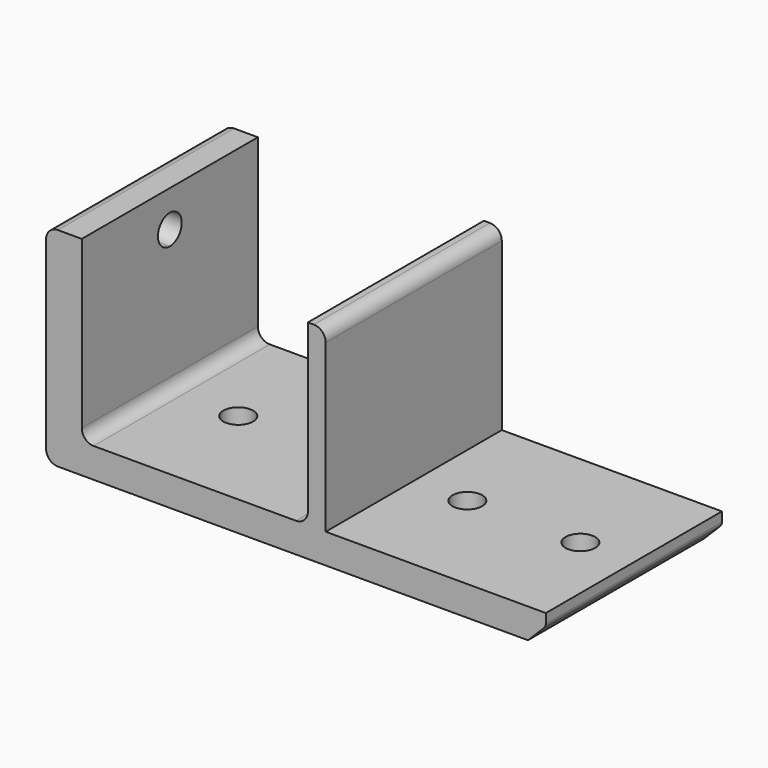
from build123d import *

# Parameters (mm, degrees)
F1_DEPTH = 35
F0_W     = 3
F0_H     = 37
F0_R     = 2.5
F0_W_2   = 37
F2_DEPTH = 5
F3_R     = 2
F4_SIZE  = 3
F5_R     = 1
F6_SIZE  = 2
F7_R     = 2
F9_DEPTH = 12.5


# Not quite as in the source:
# - a fillet or chamfer that OpenCascade refuses, or shapes differently, is made with other operations: its cross-section is extruded or revolved along the edge and cut away or added
# - a feature names something its author has since deleted; it is built from what else it names


with BuildPart() as f1:
    # F0 (on Top) → F1 (new body)
    with BuildSketch(Plane.XY):
        Polygon((-89.3438757165, 12.2090974661), (-89.3438757165, 30.7090974661), (-95.3438757165, 30.7090974661), (-95.3438757165, -6.2909025339), (-89.3438757165, -6.2909025339), align=None)
    extrude(amount=F1_DEPTH)



with BuildPart() as f1b:
    # F0 (on Top) → F1, piece 2 (new body)
    with BuildSketch(Plane.XY):
        with Locations((-49.8438757165, 12.2090974661)):
            Rectangle(F0_W, F0_H)
    extrude(amount=F1_DEPTH)


with BuildPart() as f1_1:
    add(f1.part)

    add(f1b.part)  # F2 merges F1b
    # F0 (on Top) → F2 (join)
    with BuildSketch(Plane.XY):
        Polygon((-51.3438757165, 30.7090974661), (-89.3438757165, 30.7090974661), (-89.3438757165, 12.2090974661), (-89.3438757165, -6.2909025339), (-51.3438757165, -6.2909025339), align=None)
        with Locations((-77.8438757165, 12.2090974661)):
            Circle(F0_R, mode=Mode.SUBTRACT)
        with BuildLine():
            ThreePointArc((-65.3438757165, 12.2090974661), (-62.8438757165, 14.7090974661), (-60.3438757165, 12.2090974661))
            ThreePointArc((-60.3438757165, 12.2090974661), (-62.8438757165, 9.7090974661), (-65.3438757165, 12.2090974661))
        make_face(mode=Mode.SUBTRACT)
        with Locations((-29.8438757165, 12.2090974661)):
            Rectangle(F0_W_2, F0_H)
        with Locations((-39.3354164958, 12.2090974661)):
            Circle(F0_R, mode=Mode.SUBTRACT)
        with Locations((-20.3354164958, 12.2090974661)):
            Circle(F0_R, mode=Mode.SUBTRACT)
    extrude(amount=F2_DEPTH)

    # F3
    f3_edges = [f1_1.edges().sort_by_distance(p)[0] for p in [
        (-89.343876, 12.209097, 5),
        (-51.343876, 12.209097, 5),
        (-48.343876, 12.209097, 35),
    ]]
    fillet(f3_edges, radius=F3_R)

    # F4
    f4_edges = [f1_1.edges().sort_by_distance(p)[0] for p in [
        (-11.343876, 12.209097, 0),
    ]]
    chamfer(f4_edges, length=F4_SIZE)

    # F5
    f5_edges = [f1_1.edges().sort_by_distance(p)[0] for p in [
        (-11.343876, 12.209097, 3),
    ]]
    fillet(f5_edges, radius=F5_R)

    # F6
    f6_edges = [f1_1.edges().sort_by_distance(p)[0] for p in [
        (-65.343876, 12.209097, 0),
        (-41.835416, 12.209097, 0),
        (-22.835416, 12.209097, 0),
        (-80.343876, 12.209097, 0),
    ]]
    chamfer(f6_edges, length=F6_SIZE)

    # F7
    f7_edges = [f1_1.edges().sort_by_distance(p)[0] for p in [
        (-95.343876, 12.209097, 35),
        (-95.343876, 12.209097, 0),
    ]]
    fillet(f7_edges, radius=F7_R)

    # F8 (on face) → F9 (cut, symmetric)
    with BuildSketch(Plane(origin=(-95.3438757165, 0, 0), x_dir=(0, -1, 0), z_dir=(-1, 0, 0))):
        with BuildLine():
            ThreePointArc((-9.7090974661, 28.8686309451), (-10.4413305132, 30.636397898), (-12.2090974661, 31.3686309451))
            Line((-12.2090974661, 31.3686309451), (-12.2090974661, 26.3686309451))
            ThreePointArc((-12.2090974661, 26.3686309451), (-10.4413305132, 27.1008639921), (-9.7090974661, 28.8686309451))
        make_face()
        with BuildLine():
            Line((-12.2090974661, 26.3686309451), (-12.2090974661, 31.3686309451))
            ThreePointArc((-12.2090974661, 31.3686309451), (-14.7090974661, 28.8686309451), (-12.2090974661, 26.3686309451))
        make_face()
    extrude(amount=F9_DEPTH, both=True, mode=Mode.SUBTRACT)

    # F10: chamfer of 2 on 1 edges, made by hand

    # F10_s1 → F10_t2 (revolve, cut)
    with BuildSketch(Plane.XY.offset(28.8686309451)):
        Polygon((-95.3438757165, 7.7090974661), (-93.3438757165, 9.7090974661), (-95.3438757165, 9.7090974661), align=None)
    revolve(axis=Axis((-95.3438757165, 12.2090974661, 28.8686309451), (-1, 0, 0)), mode=Mode.SUBTRACT)


solid = f1_1.part
